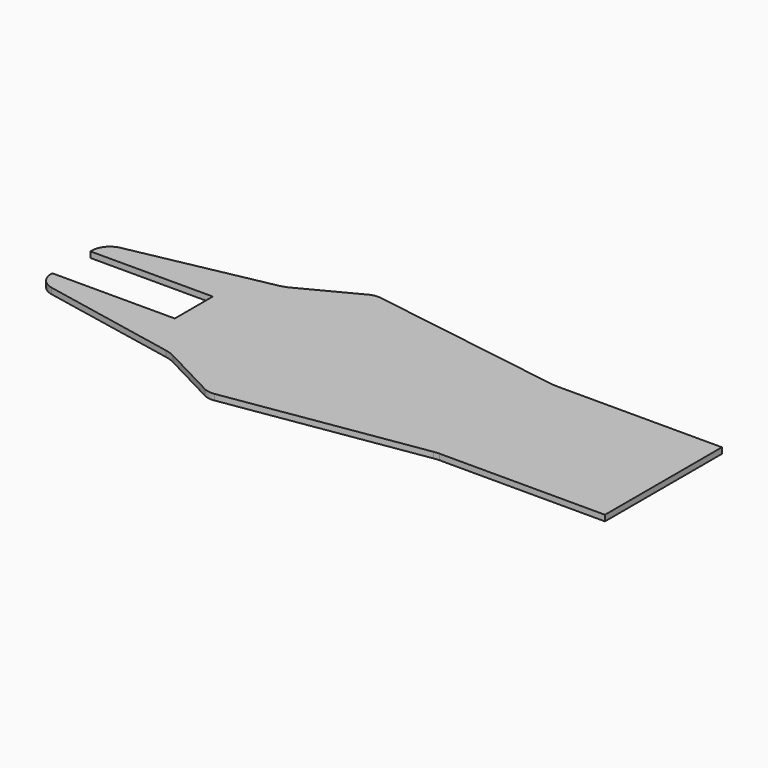
from build123d import *

# Parameters (mm, degrees)
F1_DEPTH = 8


# Not quite as in the source:
# - ends of sketch curves that miss each other by under 0.0002 mm in the source are joined


with BuildPart() as f1:
    # F0 (on Top) → F1 (new body, symmetric)
    with BuildSketch(Plane.XY):
        with BuildLine():
            Line((-475, 65), (-475, -65))
            Line((-475, -65), (-810, -65))
            Line((-810, -65), (-810, -68.972132))
            ThreePointArc((-810, -68.972132), (-798.6528240235, -100.6889917911), (-769.7616321997, -118.0099800033))
            Line((-769.7616321997, -118.0099800033), (-397.046108, -192.203936))
            ThreePointArc((-397.046108, -192.203936), (-383.3390652577, -195.9623660974), (-370.3033040103, -201.6260880198))
            Line((-370.3033040103, -201.6260880198), (-221.58307, -279.239461))
            ThreePointArc((-221.58307, -279.239461), (-206.5717643435, -284.2486537093), (-190.746885103, -284.3157393396))
            Line((-190.746885103, -284.3157393396), (342.343109, -201.193898))
            ThreePointArc((342.343109, -201.193898), (350.023164587, -200.2989211876), (357.749411, -200))
            Line((357.749411, -200), (810, -200))
            Line((810, -200), (810, 200))
            Line((810, 200), (357.749411, 200))
            ThreePointArc((357.749411, 200), (350.023164587, 200.2989211876), (342.343108949, 201.1938976727))
            Line((342.343108949, 201.1938976727), (-190.746885, 284.31574))
            ThreePointArc((-190.746885, 284.31574), (-206.5717643435, 284.2486537093), (-221.5830694776, 279.2394599991))
            Line((-221.5830694776, 279.2394599991), (-370.303304, 201.626088))
            ThreePointArc((-370.303304, 201.626088), (-383.3390652577, 195.9623660974), (-397.0461080216, 192.2039361086))
            Line((-397.0461080216, 192.2039361086), (-769.761632, 118.009979))
            ThreePointArc((-769.761632, 118.009979), (-798.6528240235, 100.6889917911), (-810, 68.972132))
            Line((-810, 68.972132), (-810, 65))
            Line((-810, 65), (-475, 65))
        make_face()
    extrude(amount=F1_DEPTH, both=True)


solid = f1.part
